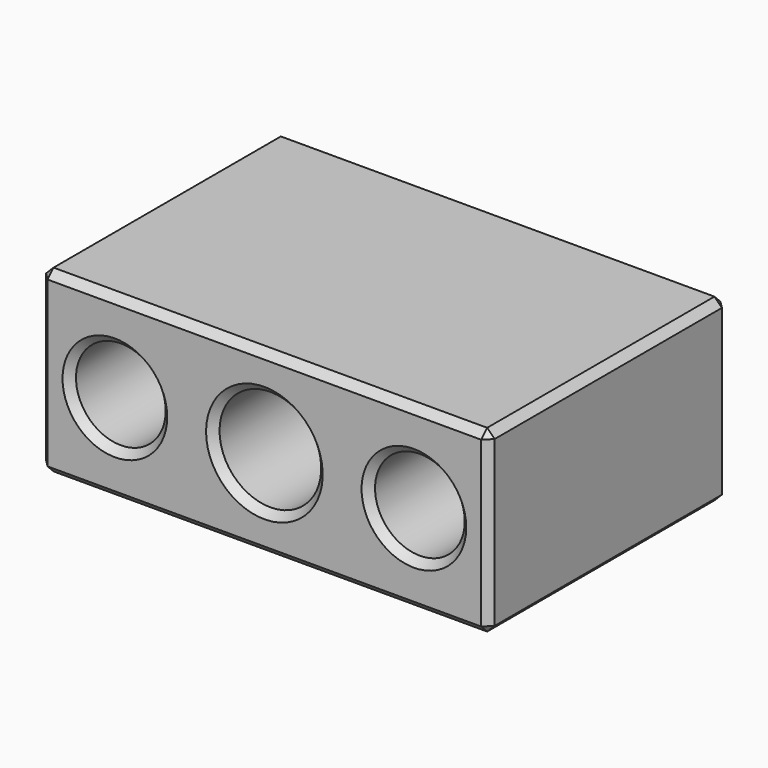
from build123d import *

# Parameters (mm, degrees)
F0_W     = 30
F0_H     = 12
F0_R     = 3
F0_R_2   = 3.4
F1_DEPTH = 20
F2_D     = 6.8
F2_DEPTH = 23.75
F2_TIP   = 2.0429261047
F3_SIZE  = 0.5


with BuildPart() as f1:
    # F0 (on Front) → F1 (new body)
    with BuildSketch(Plane.XZ):
        Rectangle(F0_W, F0_H)
        with Locations((-10, 0)):
            Circle(F0_R, mode=Mode.SUBTRACT)
        Circle(F0_R_2, mode=Mode.SUBTRACT)
        with Locations((10, 0)):
            Circle(F0_R, mode=Mode.SUBTRACT)
        Circle(F0_R_2)
    extrude(amount=F1_DEPTH)

    # F2
    with Locations(Plane(origin=(0, 0, 0), x_dir=(1, 0, 0), z_dir=(0, 1, 0))):
        with Locations((0, 0)):
            Hole(F2_D / 2, depth=F2_DEPTH)
            with Locations((0, 0, -(F2_DEPTH + F2_TIP / 2))):  # 118° drill point
                Cone(0, F2_D / 2, F2_TIP, mode=Mode.SUBTRACT)

    # F3
    f3_edges = [f1.edges().sort_by_distance(p)[0] for p in [
        (15, -10, 6),
        (-15, -10, 6),
        (0, 0, 6),
        (0, -20, 6),
        (-15, -10, -6),
        (15, -10, -6),
        (0, 0, -6),
        (0, -20, -6),
        (-15, 0, 0),
        (-15, -20, 0),
        (15, 0, 0),
        (15, -20, 0),
        (-7, -10, 0),
        (-13, 0, 0),
        (-13, -20, 0),
        (-3.4, 0, 0),
        (3.4, -10, 0),
        (-3.4, -20, 0),
        (13, -10, 0),
        (7, 0, 0),
        (7, -20, 0),
    ]]
    chamfer(f3_edges, length=F3_SIZE)


solid = f1.part
